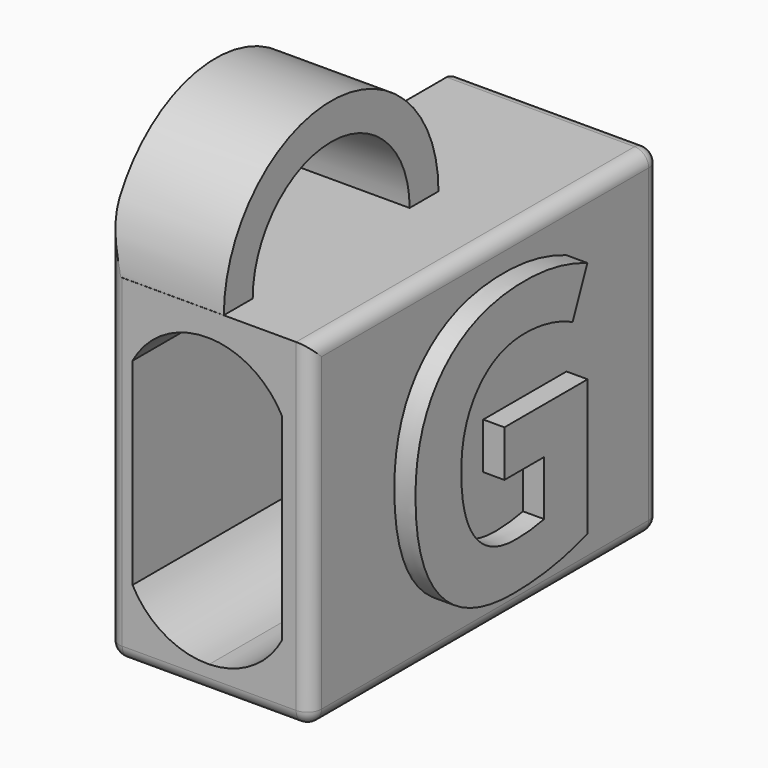
from build123d import *

# Parameters (mm, degrees)
F1_DEPTH     = 7.1664
F2_W         = 2.5832008535
F2_H         = 3.5278443415
F2_H_2       = 3.4721556585
F2_W_2       = 2.7167991465
F3_DEPTH     = 25
F4_DEPTH     = 4.1
F5_T1_DEPTH  = 14.5
F5_T3_DEPTH  = 6.1664
F5_T5_DEPTH  = 18
F5_T7_DEPTH  = 14.5
F5_T9_DEPTH  = 11
F5_T11_DEPTH = 9.6664
F5_S15_W     = 0.51
F5_S15_H     = 0.51
F5_T16_DEPTH = 0.51
F5_S21_W     = 0.51
F5_S21_H     = 0.51
F5_T22_DEPTH = 0.51
F5_S27_W     = 0.51
F5_S27_H     = 0.51
F5_T28_DEPTH = 0.51
F5_S33_W     = 0.51
F5_S33_H     = 0.51
F5_T34_DEPTH = 0.51
F5_S39_W     = 0.51
F5_S39_H     = 0.51
F5_T40_DEPTH = 0.51
F6_TEXT_SIZE = 13.0255396167
F7_DEPTH     = 0.75


# Not quite as in the source:
# - a fillet or chamfer that OpenCascade refuses, or shapes differently, is made with other operations: its cross-section is extruded or revolved along the edge and cut away or added
# - a feature names something its author has since deleted; it is built from what else it names
# - Text() gives the source's letters only with a copy of the font that has no kerning and outlines rounded to 1/6400 em; it was checked with that copy


with BuildPart() as f1:
    # F0 (on Right) → F1 (new body)
    with BuildSketch(Plane.YZ):
        with BuildLine():
            Line((7.75, 6), (1.7689648836, 6))
            ThreePointArc((1.7689648836, 6), (-2.9881978408, 1.2428372756), (-7.7453605651, 6))
            Line((-7.7453605651, 6), (-7.75, 6))
            Line((-7.75, 6), (-7.75, -6))
            Line((-7.75, -6), (7.75, -6))
            Line((7.75, -6), (7.75, 6))
        make_face()
        with BuildLine():
            Line((1.7689648836, 6), (0.4892913185, 6))
            ThreePointArc((0.4892913185, 6), (-2.9881978408, 2.5225108408), (-6.465687, 6))
            Line((-6.465687, 6), (-7.7453605651, 6))
            ThreePointArc((-7.7453605651, 6), (-2.9881978408, 1.2428372756), (1.7689648836, 6))
        make_face()
        with BuildLine():
            ThreePointArc((-6.465687, 6), (-2.9881978408, 2.5225108408), (0.4892913185, 6))
            Line((0.4892913185, 6), (-6.465687, 6))
        make_face()
    extrude(amount=F1_DEPTH)

    # F2 (on face) → F3 (cut)
    with BuildSketch(Plane(origin=(0, 7.75, 0), x_dir=(-1, 0, 0), z_dir=(0, 1, 0))):
        with BuildLine():
            Line((-3.5832, 3.5278443415), (-3.5832, 5.1208644506))
            ThreePointArc((-3.5832, 5.1208644506), (-5.0911000844, 4.6751004142), (-6.1664008535, 3.5278443415))
            Line((-6.1664008535, 3.5278443415), (-3.5832, 3.5278443415))
        make_face()
        with BuildLine():
            ThreePointArc((-0.8664008535, 3.5278443415), (-1.9989490654, 4.7095301903), (-3.5832, 5.1208644506))
            Line((-3.5832, 5.1208644506), (-3.5832, 3.5278443415))
            Line((-3.5832, 3.5278443415), (-3.5164008535, 3.5278443415))
            Line((-3.5164008535, 3.5278443415), (-0.8664008535, 3.5278443415))
        make_face()
        Polygon((-3.5164008535, 3.5278443415), (-3.5832, 3.5278443415), (-3.5832, 0), (-0.8664008535, 0), (-0.8664008535, 3.5278443415), align=None)
        with Locations((-4.8748004268, 1.7639221707)):
            Rectangle(F2_W, F2_H)
        with Locations((-4.8748004268, -1.7360778293)):
            Rectangle(F2_W, F2_H_2)
        with Locations((-2.2248004268, -1.7360778293)):
            Rectangle(F2_W_2, F2_H_2)
        with BuildLine():
            Line((-0.8664008535, -3.4721556585), (-3.5832, -3.4721556585))
            Line((-3.5832, -3.4721556585), (-3.5832, -5.0651757676))
            ThreePointArc((-3.5832, -5.0651757676), (-1.9989490654, -4.6538415074), (-0.8664008535, -3.4721556585))
        make_face()
        with BuildLine():
            Line((-3.5832, -5.0651757676), (-3.5832, -3.4721556585))
            Line((-3.5832, -3.4721556585), (-6.1664008535, -3.4721556585))
            ThreePointArc((-6.1664008535, -3.4721556585), (-5.0911000844, -4.6194117312), (-3.5832, -5.0651757676))
        make_face()
    extrude(amount=-F3_DEPTH, mode=Mode.SUBTRACT)

    # F0 (on Right) → F4 (join)
    with BuildSketch(Plane.YZ):
        with BuildLine():
            ThreePointArc((-6.465687, 6), (-2.9881978408, 9.4774891592), (0.4892913185, 6))
            Line((0.4892913185, 6), (1.7689648836, 6))
            ThreePointArc((1.7689648836, 6), (-2.9881978408, 10.7571627244), (-7.7453605651, 6))
            Line((-7.7453605651, 6), (-6.465687, 6))
        make_face()
    extrude(amount=F4_DEPTH)

    # F5: fillet of radius 0.5 on 10 edges, made by hand

    # F5_s2 → F5_t1 (cut)
    with BuildSketch(Plane.XY.offset(-5.5)):
        with BuildLine():
            ThreePointArc((6.6664, -7.75), (7.0199533906, -7.6035533906), (7.1664, -7.25))
            Line((7.1664, -7.25), (7.1764, -7.25))
            Line((7.1764, -7.25), (7.1764, -7.76))
            Line((7.1764, -7.76), (6.6664, -7.76))
            Line((6.6664, -7.76), (6.6664, -7.75))
        make_face()
        with BuildLine():
            ThreePointArc((0, -7.25), (0.1464466094, -7.6035533906), (0.5, -7.75))
            Line((0.5, -7.75), (0.5, -7.76))
            Line((0.5, -7.76), (-0.01, -7.76))
            Line((-0.01, -7.76), (-0.01, -7.25))
            Line((-0.01, -7.25), (0, -7.25))
        make_face()
        with BuildLine():
            ThreePointArc((0, 7.25), (0.1464466094, 7.6035533906), (0.5, 7.75))
            Line((0.5, 7.75), (0.5, 7.76))
            Line((0.5, 7.76), (-0.01, 7.76))
            Line((-0.01, 7.76), (-0.01, 7.25))
            Line((-0.01, 7.25), (0, 7.25))
        make_face()
    extrude(amount=F5_T1_DEPTH, mode=Mode.SUBTRACT)

    # F5_s4 → F5_t3 (cut)
    with BuildSketch(Plane.YZ.offset(0.5)):
        with BuildLine():
            ThreePointArc((-7.75, -5.5), (-7.6035533906, -5.8535533906), (-7.25, -6))
            Line((-7.25, -6), (-7.25, -6.01))
            Line((-7.25, -6.01), (-7.76, -6.01))
            Line((-7.76, -6.01), (-7.76, -5.5))
            Line((-7.76, -5.5), (-7.75, -5.5))
        make_face()
        with BuildLine():
            ThreePointArc((7.75, -5.5), (7.6035533906, -5.8535533906), (7.25, -6))
            Line((7.25, -6), (7.25, -6.01))
            Line((7.25, -6.01), (7.76, -6.01))
            Line((7.76, -6.01), (7.76, -5.5))
            Line((7.76, -5.5), (7.75, -5.5))
        make_face()
    extrude(amount=F5_T3_DEPTH, mode=Mode.SUBTRACT)

    # F5_s6 → F5_t5 (cut)
    with BuildSketch(Plane.XZ.offset(-7.25)):
        with BuildLine():
            ThreePointArc((6.6664, 6), (7.0199533906, 5.8535533906), (7.1664, 5.5))
            Line((7.1664, 5.5), (7.1764, 5.5))
            Line((7.1764, 5.5), (7.1764, 6.01))
            Line((7.1764, 6.01), (6.6664, 6.01))
            Line((6.6664, 6.01), (6.6664, 6))
        make_face()
    extrude(amount=F5_T5_DEPTH, mode=Mode.SUBTRACT)

    # F5_s8 → F5_t7 (cut)
    with BuildSketch(Plane.XZ.offset(-7.25)):
        with BuildLine():
            ThreePointArc((7.1664, -5.5), (7.0199533906, -5.8535533906), (6.6664, -6))
            Line((6.6664, -6), (6.6664, -6.01))
            Line((6.6664, -6.01), (7.1764, -6.01))
            Line((7.1764, -6.01), (7.1764, -5.5))
            Line((7.1764, -5.5), (7.1664, -5.5))
        make_face()
        with BuildLine():
            ThreePointArc((0, -5.5), (0.1464466094, -5.8535533906), (0.5, -6))
            Line((0.5, -6), (0.5, -6.01))
            Line((0.5, -6.01), (-0.01, -6.01))
            Line((-0.01, -6.01), (-0.01, -5.5))
            Line((-0.01, -5.5), (0, -5.5))
        make_face()
    extrude(amount=F5_T7_DEPTH, mode=Mode.SUBTRACT)

    # F5_s10 → F5_t9 (cut)
    with BuildSketch(Plane.XY.offset(-5.5)):
        with BuildLine():
            ThreePointArc((7.1664, 7.25), (7.0199533906, 7.6035533906), (6.6664, 7.75))
            Line((6.6664, 7.75), (6.6664, 7.76))
            Line((6.6664, 7.76), (7.1764, 7.76))
            Line((7.1764, 7.76), (7.1764, 7.25))
            Line((7.1764, 7.25), (7.1664, 7.25))
        make_face()
    extrude(amount=F5_T9_DEPTH, mode=Mode.SUBTRACT)

    # F5_s12 → F5_t11 (cut)
    with BuildSketch(Plane.YZ.offset(-3)):
        with BuildLine():
            ThreePointArc((7.25, 6), (7.6035533906, 5.8535533906), (7.75, 5.5))
            Line((7.75, 5.5), (7.76, 5.5))
            Line((7.76, 5.5), (7.76, 6.01))
            Line((7.76, 6.01), (7.25, 6.01))
            Line((7.25, 6.01), (7.25, 6))
        make_face()
    extrude(amount=F5_T11_DEPTH, mode=Mode.SUBTRACT)


with BuildPart() as f5_tool14:
    # F5_s15 → F5_t16 (new body)
    with BuildSketch(Plane.XY.offset(-5.5)):
        with Locations((6.9214, -7.505)):
            Rectangle(F5_S15_W, F5_S15_H)
    extrude(amount=-F5_T16_DEPTH)

    # F5_s17 → F5_t18 (revolve, cut)
    with BuildSketch(Plane(origin=(6.6664, -7.25, -5.5), x_dir=(-0.7071067812, 0.7071067812, 0), z_dir=(-0.7071067812, -0.7071067812, 0))):
        with BuildLine():
            ThreePointArc((0, -0.5), (0.5, 0), (0, 0.5))
            Line((0, 0.5), (0, -0.5))
        make_face()
    revolve(axis=Axis((6.6664, -7.25, -5.5), (0, 0, -1)), mode=Mode.SUBTRACT)


with BuildPart() as f1_1:
    add(f1.part)

    # F5_t13: cut F5_tool14
    add(f5_tool14.part, mode=Mode.SUBTRACT)


with BuildPart() as f5_tool20:
    # F5_s21 → F5_t22 (new body)
    with BuildSketch(Plane.XY.offset(-5.5)):
        with Locations((0.245, -7.505)):
            Rectangle(F5_S21_W, F5_S21_H)
    extrude(amount=-F5_T22_DEPTH)

    # F5_s23 → F5_t24 (revolve, cut)
    with BuildSketch(Plane(origin=(0.5, -7.25, -5.5), x_dir=(0.7071067812, 0.7071067812, 0), z_dir=(-0.7071067812, 0.7071067812, 0))):
        with BuildLine():
            ThreePointArc((0, -0.5), (0.5, 0), (0, 0.5))
            Line((0, 0.5), (0, -0.5))
        make_face()
    revolve(axis=Axis((0.5, -7.25, -5.5), (0, 0, -1)), mode=Mode.SUBTRACT)


with BuildPart() as f1_2:
    add(f1_1.part)

    # F5_t19: cut F5_tool20
    add(f5_tool20.part, mode=Mode.SUBTRACT)


with BuildPart() as f5_tool26:
    # F5_s27 → F5_t28 (new body)
    with BuildSketch(Plane.XY.offset(5.5)):
        with Locations((6.9214, 7.505)):
            Rectangle(F5_S27_W, F5_S27_H)
    extrude(amount=F5_T28_DEPTH)

    # F5_s29 → F5_t30 (revolve, cut)
    with BuildSketch(Plane(origin=(6.6664, 7.25, 5.5), x_dir=(-0.7071067812, -0.7071067812, 0), z_dir=(-0.7071067812, 0.7071067812, 0))):
        with BuildLine():
            ThreePointArc((0, -0.5), (0.5, 0), (0, 0.5))
            Line((0, 0.5), (0, -0.5))
        make_face()
    revolve(axis=Axis((6.6664, 7.25, 5.5), (0, 0, 1)), mode=Mode.SUBTRACT)


with BuildPart() as f1_3:
    add(f1_2.part)

    # F5_t25: cut F5_tool26
    add(f5_tool26.part, mode=Mode.SUBTRACT)


with BuildPart() as f5_tool32:
    # F5_s33 → F5_t34 (new body)
    with BuildSketch(Plane.XY.offset(-5.5)):
        with Locations((6.9214, 7.505)):
            Rectangle(F5_S33_W, F5_S33_H)
    extrude(amount=-F5_T34_DEPTH)

    # F5_s35 → F5_t36 (revolve, cut)
    with BuildSketch(Plane(origin=(6.6664, 7.25, -5.5), x_dir=(-0.7071067812, -0.7071067812, 0), z_dir=(0.7071067812, -0.7071067812, 0))):
        with BuildLine():
            ThreePointArc((0, -0.5), (0.5, 0), (0, 0.5))
            Line((0, 0.5), (0, -0.5))
        make_face()
    revolve(axis=Axis((6.6664, 7.25, -5.5), (0, 0, -1)), mode=Mode.SUBTRACT)


with BuildPart() as f1_4:
    add(f1_3.part)

    # F5_t31: cut F5_tool32
    add(f5_tool32.part, mode=Mode.SUBTRACT)


with BuildPart() as f5_tool38:
    # F5_s39 → F5_t40 (new body)
    with BuildSketch(Plane.XY.offset(-5.5)):
        with Locations((0.245, 7.505)):
            Rectangle(F5_S39_W, F5_S39_H)
    extrude(amount=-F5_T40_DEPTH)

    # F5_s41 → F5_t42 (revolve, cut)
    with BuildSketch(Plane(origin=(0.5, 7.25, -5.5), x_dir=(0.7071067812, -0.7071067812, 0), z_dir=(0.7071067812, 0.7071067812, 0))):
        with BuildLine():
            ThreePointArc((0, -0.5), (0.5, 0), (0, 0.5))
            Line((0, 0.5), (0, -0.5))
        make_face()
    revolve(axis=Axis((0.5, 7.25, -5.5), (0, 0, -1)), mode=Mode.SUBTRACT)


with BuildPart() as f1_5:
    add(f1_4.part)

    # F5_t37: cut F5_tool38
    add(f5_tool38.part, mode=Mode.SUBTRACT)

    # F6 (on face) → F7 (join)
    with BuildSketch(Plane.YZ.offset(7.1664)):
        with Locations((-4.7791411635, -4.5978116977)):
            Text('G', F6_TEXT_SIZE, font='Open Sans', font_style=FontStyle.BOLD, text_align=(TextAlign.LEFT, TextAlign.BOTTOM))
    extrude(amount=F7_DEPTH)


solid = f1_5.part
